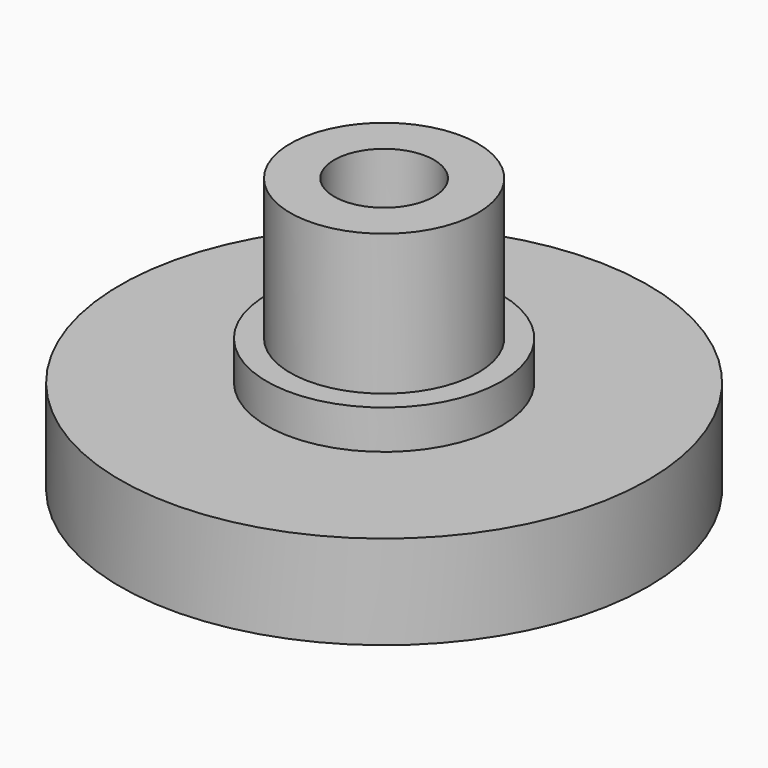
from build123d import *

# Parameters (mm, degrees)
F0_R      = 8.9296875
F0_R_2    = 3.96875
F0_R_3    = 3.175
F0_R_4    = 1.68671875
F1_DEPTH  = 3.175
F2_DEPTH  = 1.3208
F3_DEPTH  = 6.0833
F1_FACE_R = 8.9296875


# Not quite as in the source:
# - a length typed as a fraction of an inch, garbled in the dataset ("3 / 203.2 mm" for 3/8 in), is restored


with BuildPart() as f1:
    # F0 (on Top) → F1 (new body)
    with BuildSketch(Plane.XY):
        Circle(F0_R)
        Circle(F0_R_2, mode=Mode.SUBTRACT)
        Circle(F0_R_2)
        Circle(F0_R_3, mode=Mode.SUBTRACT)
        Circle(F0_R_3)
        Circle(F0_R_4, mode=Mode.SUBTRACT)
        Circle(F0_R_4)
    extrude(amount=-F1_DEPTH)

    # F0 (on Top) → F2 (join)
    with BuildSketch(Plane.XY):
        Circle(F0_R_2)
        Circle(F0_R_3, mode=Mode.SUBTRACT)
        Circle(F0_R_3)
        Circle(F0_R_4, mode=Mode.SUBTRACT)
        Circle(F0_R_4)
    extrude(amount=F2_DEPTH)

    # F0 (on Top) → F3 (join)
    with BuildSketch(Plane.XY):
        Circle(F0_R_3)
        Circle(F0_R_4, mode=Mode.SUBTRACT)
    extrude(amount=F3_DEPTH)

    # F1_face (on face) → F4 section 0
    with BuildSketch(Plane(origin=(0, 0, -3.175), x_dir=(1, 0, 0), z_dir=(0, 0, -1)), mode=Mode.PRIVATE) as f4_s0:
        Circle(F1_FACE_R)
    loft([f4_s0.sketch, Vertex(0, 0, 0)], mode=Mode.SUBTRACT)


solid = f1.part
